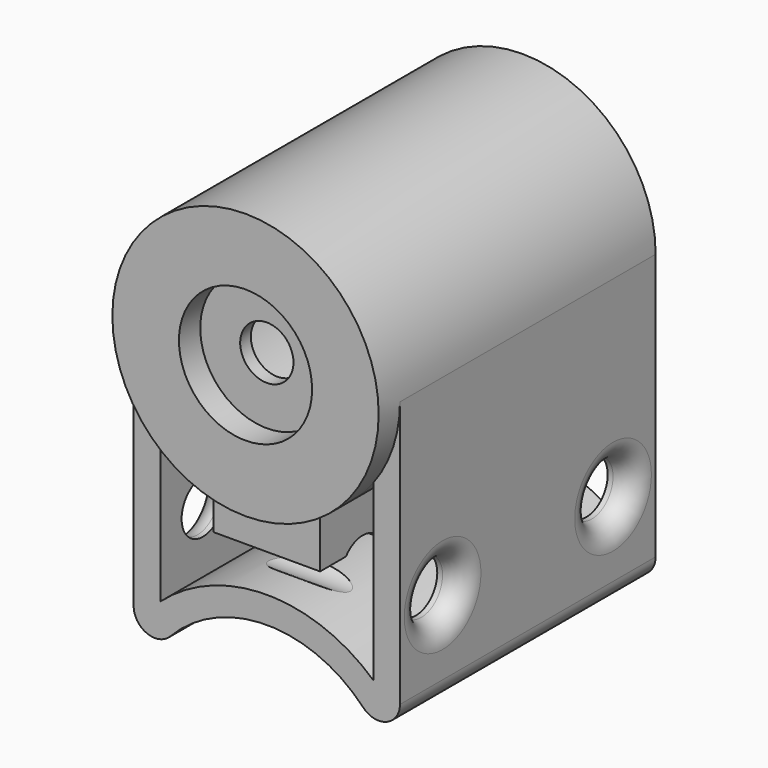
from build123d import *

# Parameters (mm, degrees)
F1_DEPTH = 38.1
F2_R     = 3.175
F3_DEPTH = 25.4
F4_R     = 2.53999
F5_R     = 2.54
F6_R     = 3.175
F7_DEPTH = 1.5875
F8_R     = 15.875
F8_R_2   = 7.9375
F9_DEPTH = 3.175


# Not quite as in the source:
# - a fillet or chamfer is up to 0.001 mm smaller than in the source, because OpenCascade refuses the exact size
# - a feature names something its author has since deleted; it is built from what else it names


with BuildPart() as f1:
    # F0 (on Front) → F1 (new body)
    with BuildSketch(Plane.XZ):
        with BuildLine():
            ThreePointArc((-15.875, -44.45), (0, -28.575), (15.875, -44.45))
            Line((15.875, -44.45), (15.875, 0))
            ThreePointArc((15.875, 0), (15.0603473566, -5.0201157855), (12.7, -9.525))
            Line((12.7, -9.525), (12.7, -30.2509683429))
            ThreePointArc((12.7, -30.2509683429), (0, -25.4), (-12.7, -30.2509683429))
            Line((-12.7, -30.2509683429), (-12.7, -9.525))
            ThreePointArc((-12.7, -9.525), (-15.0603473566, -5.0201157855), (-15.875, 0))
            Line((-15.875, 0), (-15.875, -44.45))
        make_face()
        with BuildLine():
            ThreePointArc((12.7, -9.525), (15.0603473566, -5.0201157855), (15.875, 0))
            ThreePointArc((15.875, 0), (0, 15.875), (-15.875, 0))
            ThreePointArc((-15.875, 0), (-15.0603473566, -5.0201157855), (-12.7, -9.525))
            ThreePointArc((-12.7, -9.525), (-9.8507599619, -12.4490221774), (-6.35, -14.5496778315))
            Line((-6.35, -14.5496778315), (-6.35, -20.8996778315))
            Line((-6.35, -20.8996778315), (6.35, -20.8996778315))
            Line((6.35, -20.8996778315), (6.35, -14.5496778315))
            ThreePointArc((6.35, -14.5496778315), (9.8507599619, -12.4490221774), (12.7, -9.525))
        make_face()
        with BuildLine():
            Line((-3.175, -18.6467221242), (-3.175, -12.2967221242))
            ThreePointArc((-3.175, -12.2967221242), (0, 12.7), (3.175, -12.2967221242))
            Line((3.175, -12.2967221242), (3.175, -18.6467221242))
            Line((3.175, -18.6467221242), (-3.175, -18.6467221242))
        make_face(mode=Mode.SUBTRACT)
    extrude(amount=F1_DEPTH)

    # F2 (on Right) → F3 (cut, symmetric)
    with BuildSketch(Plane.YZ):
        with Locations((-31.75, -22.86)):
            Circle(F2_R)
        with Locations((-6.35, -22.86)):
            Circle(F2_R)
    extrude(amount=F3_DEPTH, both=True, mode=Mode.SUBTRACT)

    # F4 (radius 2.54 in the source; OpenCascade refuses exactly that, so slightly less here)
    f4_edges = [f1.edges().sort_by_distance(p)[0] for p in [
        (15.875, -19.05, -44.45),
        (-15.875, -19.05, -44.45),
    ]]
    fillet(f4_edges, radius=F4_R)

    # F5
    f5_edges = [f1.edges().sort_by_distance(p)[0] for p in [
        (-15.875, -9.525, -22.86),
        (-15.875, -34.925, -22.86),
        (15.875, -34.925, -22.86),
        (15.875, -9.525, -22.86),
    ]]
    fillet(f5_edges, radius=F5_R)

    # F6 (on face) → F7 (join)
    with BuildSketch(Plane.XZ.offset(38.1)):
        with BuildLine():
            ThreePointArc((6.35, -14.5496778315), (0, 15.875), (-6.35, -14.5496778315))
            Line((-6.35, -14.5496778315), (-6.35, -20.8996778315))
            Line((-6.35, -20.8996778315), (6.35, -20.8996778315))
            Line((6.35, -20.8996778315), (6.35, -14.5496778315))
        make_face()
        Circle(F6_R, mode=Mode.SUBTRACT)
    extrude(amount=-F7_DEPTH)

    # F8 (on face) → F9 (join)
    with BuildSketch(Plane.XZ.offset(38.1)):
        Circle(F8_R)
        Circle(F8_R_2, mode=Mode.SUBTRACT)
    extrude(amount=F9_DEPTH)


solid = f1.part
